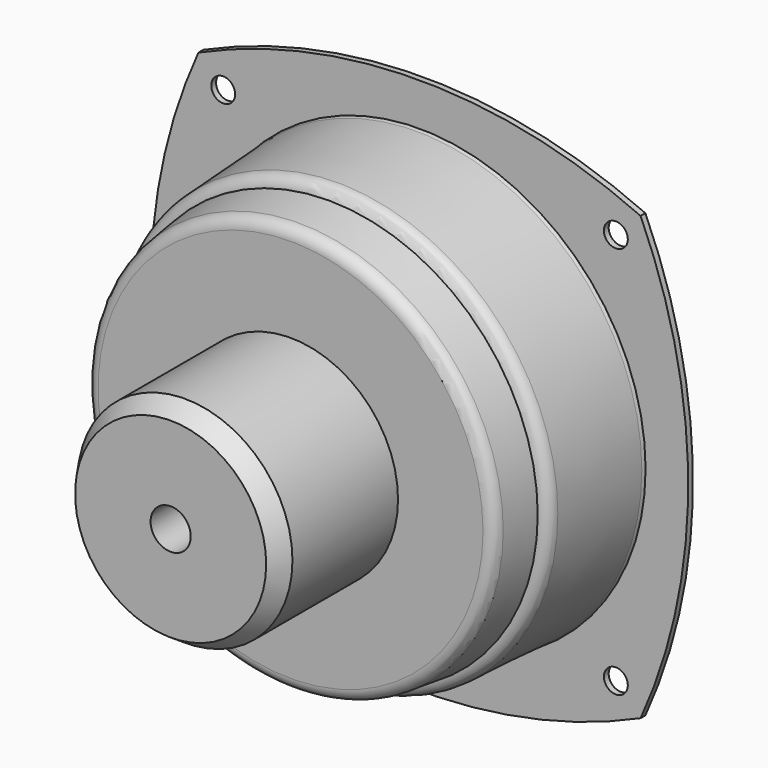
from build123d import *

# Parameters (mm, degrees)
F1_DEPTH  = 1
F2_R      = 37.75
F3_DEPTH  = 19
F4_SIZE2  = 18.99999
F4_SIZE   = 0.99999
F5_R      = 35
F6_DEPTH  = 8
F7_SIZE2  = 7.99999
F7_SIZE   = 0.99999
F9_R      = 2
F10_R     = 18
F11_DEPTH = 25.1
F12_SIZE2 = 3
F12_SIZE  = 2
F13_R     = 3.3621070756
F14_DEPTH = 25
F15_R     = 2
F16_DEPTH = 53.101
F19_R     = 6.5


# Not quite as in the source:
# - a fillet or chamfer that OpenCascade refuses, or shapes differently, is made with other operations: its cross-section is extruded or revolved along the edge and cut away or added
# - a fillet or chamfer is up to 0.001 mm smaller than in the source, because OpenCascade refuses the exact size


with BuildPart() as f1:
    # F0 (on Front) → F1 (new body)
    with BuildSketch(Plane.XZ):
        with BuildLine():
            ThreePointArc((37.029404499, -37.029404499), (45, 0), (37.029404499, 37.029404499))
            ThreePointArc((37.029404499, 37.029404499), (0, 45), (-37.029404499, 37.029404499))
            ThreePointArc((-37.029404499, 37.029404499), (-45, 0), (-37.029404499, -37.029404499))
            ThreePointArc((-37.029404499, -37.029404499), (0, -45), (37.029404499, -37.029404499))
        make_face()
    extrude(amount=F1_DEPTH)

    # F2 (on face) → F3 (join)
    with BuildSketch(Plane.XZ.offset(1)):
        Circle(F2_R)
    extrude(amount=F3_DEPTH)

    # F4 (size 1 and 19 in the source; OpenCascade refuses exactly that, so slightly less here)
    f4_edges = [f1.edges().sort_by_distance(p)[0] for p in [
        (-37.75, -20, 0),
    ]]
    f4_side = f1.faces().sort_by_distance((0, -20, 0))[0]
    chamfer(f4_edges, length=F4_SIZE, length2=F4_SIZE2, reference=f4_side)

    # F5 (on face) → F6 (join)
    with BuildSketch(Plane.XZ.offset(20)):
        Circle(F5_R)
    extrude(amount=F6_DEPTH)

    # F7 (size 1 and 8 in the source; OpenCascade refuses exactly that, so slightly less here)
    f7_edges = [f1.edges().sort_by_distance(p)[0] for p in [
        (-35, -28, 0),
    ]]
    f7_side = f1.faces().sort_by_distance((0, -28, 0))[0]
    chamfer(f7_edges, length=F7_SIZE, length2=F7_SIZE2, reference=f7_side)

    # F8: fillet of radius 2 on 1 edges, made by hand

    # F8_s1 → F8_t2 (revolve, cut)
    with BuildSketch(Plane.XY):
        with BuildLine():
            ThreePointArc((35, -20), (36.2814643906, -19.4044849409), (36.8494519972, -18.110584153))
            Line((36.8494519972, -18.110584153), (36.8893967114, -18.1126864865))
            Line((36.8893967114, -18.1126864865), (36.7899547142, -20.0021023335))
            Line((36.7899547142, -20.0021023335), (36.75001, -20.04))
            ThreePointArc((36.75001, -20.04), (35.875005, -20.04), (35.0029556743, -20.0398906504))
            Line((35.0029556743, -20.0398906504), (35, -20))
        make_face()
    revolve(axis=Axis((0, -20, 0), (0, -1, 0)), mode=Mode.SUBTRACT)

    # F9
    f9_edges = [f1.edges().sort_by_distance(p)[0] for p in [
        (-34.00001, -28, 0),
    ]]
    fillet(f9_edges, radius=F9_R)

    # F10 (on face) → F11 (join)
    with BuildSketch(Plane.XZ.offset(28)):
        Circle(F10_R)
    extrude(amount=F11_DEPTH)

    # F12
    f12_edges = [f1.edges().sort_by_distance(p)[0] for p in [
        (-18, -53.1, 0),
    ]]
    f12_side = f1.faces().sort_by_distance((0, -53.1, 0))[0]
    chamfer(f12_edges, length=F12_SIZE, length2=F12_SIZE2, reference=f12_side)

    # F13 (on face) → F14 (cut)
    with BuildSketch(Plane.XZ.offset(53.1)):
        Circle(F13_R)
    extrude(amount=-F14_DEPTH, mode=Mode.SUBTRACT)

    # F15 (on face) → F16 (cut, through all)
    with BuildSketch(Plane(origin=(0, 0, 0), x_dir=(-1, 0, 0), z_dir=(0, 1, 0))):
        with Locations((-32.8804653252, 32.8804653252)):
            Circle(F15_R)
        with Locations((-32.8804653252, -32.8804653252)):
            Circle(F15_R)
        with Locations((32.8804653252, -32.8804653252)):
            Circle(F15_R)
        with Locations((32.8804653252, 32.8804653252)):
            Circle(F15_R)
    extrude(amount=-F16_DEPTH, mode=Mode.SUBTRACT)

    # F17 (on Top) → F18 (revolve, cut)
    with BuildSketch(Plane.XY):
        with BuildLine():
            Line((0, 0), (-25, 0))
            ThreePointArc((-25, 0), (-13.3392655896, -6.9096080905), (0, -9.3136472921))
            Line((0, -9.3136472921), (0, 0))
        make_face()
    revolve(axis=Axis((0, 14.4480448216, 0), (0, 1, 0)), mode=Mode.SUBTRACT)

    # F19 (on Top) → F20 (revolve)
    with BuildSketch(Plane.XY):
        with Locations((-31.4735865454, 0.2)):
            Circle(F19_R)
    revolve(axis=Axis((0, 14.4480448216, 0), (0, 1, 0)))


solid = f1.part
